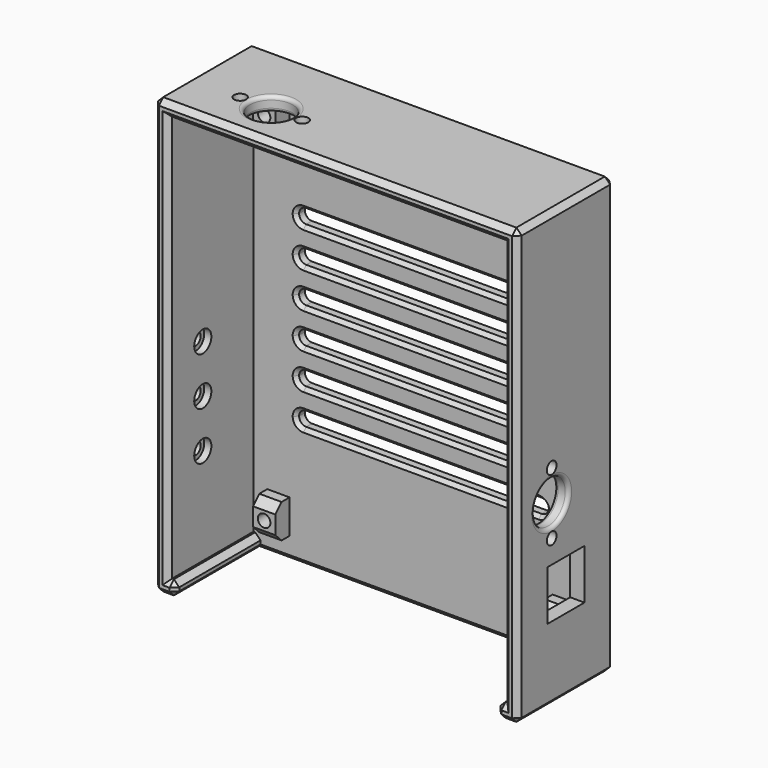
from build123d import *

# Parameters (mm, degrees)
F0_W      = 6.25
F0_H      = 9.5
F0_W_2    = 70
F0_H_2    = 4
F0_W_3    = 90
F1_DEPTH  = 4
F0_R      = 1.75
F2_DEPTH  = 9
F3_SIZE   = 2.2
F4_R      = 1.99999
F5_DEPTH  = 34
F6_DEPTH  = 4
F7_W      = 13
F7_H      = 14
F7_R      = 6
F7_R_2    = 1.7
F8_DEPTH  = 5
F9_R      = 6
F9_R_2    = 1.7
F10_DEPTH = 5
F11_SIZE  = 1.5
F12_SIZE  = 1
F13_R     = 0.99999
F14_R     = 1.75
F15_DEPTH = 5
F14_R_2   = 3
F16_DEPTH = 2


# Not quite as in the source:
# - a fillet or chamfer is up to 0.001 mm smaller than in the source, because OpenCascade refuses the exact size


with BuildPart() as f1:
    # F0 (on Front) → F1 (new body)
    with BuildSketch(Plane.XZ):
        Polygon((-45, -57), (45, -57), (47, -57), (47, 57), (-47, 57), (-47, -57), align=None)
        with Locations((-40, -50)):
            Rectangle(F0_W, F0_H, mode=Mode.SUBTRACT)
        with Locations((40, -50)):
            Rectangle(F0_W, F0_H, mode=Mode.SUBTRACT)
        with Locations((0, -25)):
            Rectangle(F0_W_2, F0_H_2, mode=Mode.SUBTRACT)
        with Locations((0, -15)):
            Rectangle(F0_W_2, F0_H_2, mode=Mode.SUBTRACT)
        with Locations((0, -5)):
            Rectangle(F0_W_2, F0_H_2, mode=Mode.SUBTRACT)
        with Locations((-40, 50)):
            Rectangle(F0_W, F0_H, mode=Mode.SUBTRACT)
        with Locations((0, 5)):
            Rectangle(F0_W_2, F0_H_2, mode=Mode.SUBTRACT)
        with Locations((0, 15)):
            Rectangle(F0_W_2, F0_H_2, mode=Mode.SUBTRACT)
        with Locations((0, 25)):
            Rectangle(F0_W_2, F0_H_2, mode=Mode.SUBTRACT)
        with Locations((40, 50)):
            Rectangle(F0_W, F0_H, mode=Mode.SUBTRACT)
        with Locations((0, -59)):
            Rectangle(F0_W_3, F0_H_2)
    extrude(amount=F1_DEPTH)

    # F0 (on Front) → F2 (join)
    with BuildSketch(Plane.XZ):
        with Locations((40, -50)):
            Rectangle(F0_W, F0_H)
        Polygon((40, -46.4492958445), (43.075, -48.2246479222), (43.075, -51.7753520778), (40, -53.5507041555), (36.925, -51.7753520778), (36.925, -48.2246479222), align=None, mode=Mode.SUBTRACT)
        with Locations((-40, -50)):
            Rectangle(F0_W, F0_H)
        Polygon((-40, -46.4492958445), (-36.925, -48.2246479222), (-36.925, -51.7753520778), (-40, -53.5507041555), (-43.075, -51.7753520778), (-43.075, -48.2246479222), align=None, mode=Mode.SUBTRACT)
        with Locations((-40, 50)):
            Rectangle(F0_W, F0_H)
        Polygon((-40, 53.5507041555), (-36.925, 51.7753520778), (-36.925, 48.2246479222), (-40, 46.4492958445), (-43.075, 48.2246479222), (-43.075, 51.7753520778), align=None, mode=Mode.SUBTRACT)
        with Locations((40, 50)):
            Rectangle(F0_W, F0_H)
        Polygon((40, 46.4492958445), (36.925, 48.2246479222), (36.925, 51.7753520778), (40, 53.5507041555), (43.075, 51.7753520778), (43.075, 48.2246479222), align=None, mode=Mode.SUBTRACT)
        Polygon((-36.925, -51.7753520778), (-36.925, -48.2246479222), (-40, -46.4492958445), (-43.075, -48.2246479222), (-43.075, -51.7753520778), (-40, -53.5507041555), align=None)
        with Locations((-40, -50)):
            Circle(F0_R, mode=Mode.SUBTRACT)
        Polygon((43.075, -51.7753520778), (43.075, -48.2246479222), (40, -46.4492958445), (36.925, -48.2246479222), (36.925, -51.7753520778), (40, -53.5507041555), align=None)
        with Locations((40, -50)):
            Circle(F0_R, mode=Mode.SUBTRACT)
        Polygon((36.925, 51.7753520778), (36.925, 48.2246479222), (40, 46.4492958445), (43.075, 48.2246479222), (43.075, 51.7753520778), (40, 53.5507041555), align=None)
        with Locations((40, 50)):
            Circle(F0_R, mode=Mode.SUBTRACT)
        Polygon((-36.925, 48.2246479222), (-36.925, 51.7753520778), (-40, 53.5507041555), (-43.075, 51.7753520778), (-43.075, 48.2246479222), (-40, 46.4492958445), align=None)
        with Locations((-40, 50)):
            Circle(F0_R, mode=Mode.SUBTRACT)
    extrude(amount=F2_DEPTH)

    # F3
    f3_edges = [f1.edges().sort_by_distance(p)[0] for p in [
        (-40, -9, -45.25),
        (-40, -9, -54.75),
        (40, -9, -45.25),
        (40, -9, -54.75),
        (-40, -9, 54.75),
        (-40, -9, 45.25),
        (40, -9, 54.75),
        (40, -9, 45.25),
    ]]
    chamfer(f3_edges, length=F3_SIZE)

    # F4 (radius 2 in the source; OpenCascade refuses exactly that, so slightly less here)
    f4_edges = [f1.edges().sort_by_distance(p)[0] for p in [
        (35, -2, -27),
        (35, -2, -23),
        (35, -2, -13),
        (35, -2, -3),
        (35, -2, 7),
        (35, -2, 17),
        (35, -2, 27),
        (-35, -2, 27),
        (-35, -2, 17),
        (-35, -2, 7),
        (-35, -2, -3),
        (-35, -2, -13),
        (-35, -2, -23),
        (35, -2, -17),
        (35, -2, -7),
        (35, -2, 3),
        (35, -2, 13),
        (35, -2, 23),
        (-35, -2, 23),
        (-35, -2, 13),
        (-35, -2, 3),
        (-35, -2, -7),
        (-35, -2, -17),
        (-35, -2, -27),
    ]]
    fillet(f4_edges, radius=F4_R)

    # F0 (on Front) → F5 (join)
    with BuildSketch(Plane.XZ):
        Polygon((45, -61), (51, -61), (51, 61), (-51, 61), (-51, -61), (-45, -61), (-45, -57), (-47, -57), (-47, 57), (47, 57), (47, -57), (45, -57), align=None)
    extrude(amount=F5_DEPTH)

    # F0 (on Front) → F6 (cut)
    with BuildSketch(Plane.XZ):
        Polygon((36.925, 51.7753520778), (36.925, 48.2246479222), (40, 46.4492958445), (43.075, 48.2246479222), (43.075, 51.7753520778), (40, 53.5507041555), align=None)
        with Locations((40, 50)):
            Circle(F0_R, mode=Mode.SUBTRACT)
        Polygon((-36.925, 48.2246479222), (-36.925, 51.7753520778), (-40, 53.5507041555), (-43.075, 51.7753520778), (-43.075, 48.2246479222), (-40, 46.4492958445), align=None)
        with Locations((-40, 50)):
            Circle(F0_R, mode=Mode.SUBTRACT)
        Polygon((43.075, -51.7753520778), (43.075, -48.2246479222), (40, -46.4492958445), (36.925, -48.2246479222), (36.925, -51.7753520778), (40, -53.5507041555), align=None)
        with Locations((40, -50)):
            Circle(F0_R, mode=Mode.SUBTRACT)
        Polygon((-36.925, -51.7753520778), (-36.925, -48.2246479222), (-40, -46.4492958445), (-43.075, -48.2246479222), (-43.075, -51.7753520778), (-40, -53.5507041555), align=None)
        with Locations((-40, -50)):
            Circle(F0_R, mode=Mode.SUBTRACT)
    extrude(amount=F6_DEPTH, mode=Mode.SUBTRACT)

    # F7 (on face) → F8 (cut)
    with BuildSketch(Plane(origin=(47, 0, 0), x_dir=(0, -1, 0), z_dir=(-1, 0, 0))):
        with Locations((17, -33)):
            Rectangle(F7_W, F7_H)
        with Locations((22, -10.7700689131)):
            Circle(F7_R)
        with Locations((22, -19.4700689131)):
            Circle(F7_R_2)
        with Locations((22, -2.0700689131)):
            Circle(F7_R_2)
    extrude(amount=-F8_DEPTH, mode=Mode.SUBTRACT)

    # F9 (on face) → F10 (cut)
    with BuildSketch(Plane.XY.offset(61)):
        with Locations((-27.6179584248, -22)):
            Circle(F9_R)
        with Locations((-36.3179584248, -22)):
            Circle(F9_R_2)
        with Locations((-18.9179584248, -22)):
            Circle(F9_R_2)
    extrude(amount=-F10_DEPTH, mode=Mode.SUBTRACT)

    # F11
    f11_edges = [f1.edges().sort_by_distance(p)[0] for p in [
        (51, 0, 0),
        (51, -17, 61),
        (51, -34, 0),
        (0, -34, 61),
        (0, 0, 61),
        (-51, 0, 0),
        (-51, -17, 61),
        (-51, -34, 0),
        (-51, -17, -61),
        (0, 0, -61),
        (51, -17, -61),
        (45, -19, -61),
        (48, -34, -61),
        (-48, -34, -61),
        (47, -34, 0),
        (0, -34, 57),
        (-47, -34, 0),
        (46, -34, -57),
        (45, -34, -59),
        (-46, -34, -57),
        (-45, -19, -57),
        (-45, -19, -61),
        (-45, -34, -59),
        (0, -4, -61),
        (45, -19, -57),
    ]]
    chamfer(f11_edges, length=F11_SIZE)

    # F12
    f12_edges = [f1.edges().sort_by_distance(p)[0] for p in [
        (0, -4, -27),
        (-34.414216, -4, -23.585784),
        (0, -4, -23),
        (34.414216, -4, -26.414216),
        (34.414216, -4, -16.414216),
        (0, -4, -17),
        (0, -4, -13),
        (-34.414216, -4, -13.585784),
        (0, -4, -7),
        (-34.414216, -4, -3.585784),
        (34.414216, -4, -6.414216),
        (0, -4, -3),
        (0, -4, 3),
        (34.414216, -4, 3.585784),
        (0, -4, 7),
        (-34.414216, -4, 6.414216),
        (0, -4, 13),
        (-34.414216, -4, 16.414216),
        (34.414216, -4, 13.585784),
        (0, -4, 17),
        (0, -4, 23),
        (34.414216, -4, 23.585784),
        (0, -4, 27),
        (-34.414216, -4, 26.414216),
        (0, 0, -27),
        (34.414216, 0, -26.414216),
        (0, 0, -23),
        (-34.414216, 0, -23.585784),
        (-34.414216, 0, -13.585784),
        (0, 0, -17),
        (34.414216, 0, -16.414216),
        (0, 0, -13),
        (0, 0, -7),
        (34.414216, 0, -6.414216),
        (0, 0, -3),
        (-34.414216, 0, -3.585784),
        (-34.414216, 0, 6.414216),
        (0, 0, 3),
        (0, 0, 7),
        (34.414216, 0, 3.585784),
        (0, 0, 13),
        (34.414216, 0, 13.585784),
        (0, 0, 17),
        (-34.414216, 0, 16.414216),
        (0, 0, 23),
        (-34.414216, 0, 26.414216),
        (0, 0, 27),
        (34.414216, 0, 23.585784),
    ]]
    chamfer(f12_edges, length=F12_SIZE)

    # F13 (radius 1 in the source; OpenCascade refuses exactly that, so slightly less here)
    f13_edges = [f1.edges().sort_by_distance(p)[0] for p in [
        (51, -16, -10.770069),
        (47, -16, -10.770069),
        (-33.617958, -22, 61),
        (-33.617958, -22, 57),
    ]]
    fillet(f13_edges, radius=F13_R)

    # F14 (on face) → F15 (cut)
    with BuildSketch(Plane.YZ.offset(-47)):
        with Locations((-21.75, -2.85)):
            Circle(F14_R)
        with Locations((-21.75, -16.35)):
            Circle(F14_R)
        with Locations((-21.75, -29.85)):
            Circle(F14_R)
    extrude(amount=-F15_DEPTH, mode=Mode.SUBTRACT)

    # F14 (on face) → F16 (cut)
    with BuildSketch(Plane.YZ.offset(-47)):
        with Locations((-21.75, -29.85)):
            Circle(F14_R_2)
        with Locations((-21.75, -29.85)):
            Circle(F14_R, mode=Mode.SUBTRACT)
        with Locations((-21.75, -16.35)):
            Circle(F14_R_2)
        with Locations((-21.75, -16.35)):
            Circle(F14_R, mode=Mode.SUBTRACT)
        with Locations((-21.75, -2.85)):
            Circle(F14_R_2)
        with Locations((-21.75, -2.85)):
            Circle(F14_R, mode=Mode.SUBTRACT)
    extrude(amount=-F16_DEPTH, mode=Mode.SUBTRACT)


solid = f1.part
